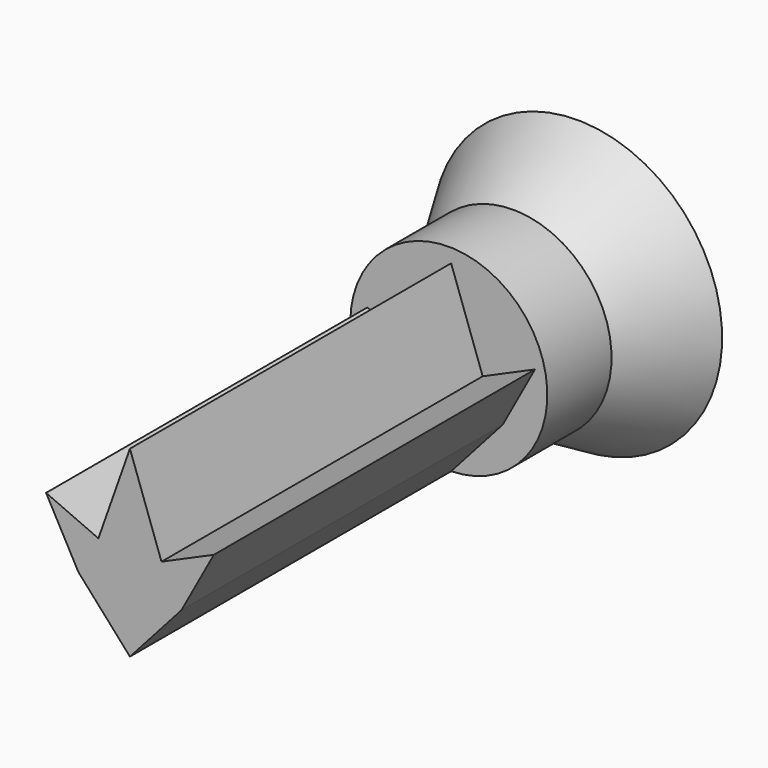
from build123d import *

# Parameters (mm, degrees)
F1_DEPTH  = 75
F3_DEPTH  = 15
F3_FACE_R = 18.3992120147
F4_DEPTH  = 15
F4_TAPER  = -30


with BuildPart() as f1:
    # F0 (on Front) → F1 (new body)
    with BuildSketch(Plane.XZ):
        Polygon((-15.2326680545, 3.4489048412), (-9.1970840294, -7.6163323829), (0.4311103548, -18.3941606665), (10.0593047391, -7.6163323829), (16.0948887642, 3.4489048412), (6.3229899097, -0.8622264722), (0.4311103548, 15.8074827632), (-5.4607692, -0.8622264722), align=None)
    extrude(amount=F1_DEPTH)


with BuildPart() as f3:
    # F2 (on face) → F3 (new body)
    with BuildSketch(Plane(origin=(0, 0, 0), x_dir=(-1, 0, 0), z_dir=(0, 1, 0))):
        with BuildLine():
            ThreePointArc((-0.4311103548, -18.3941606665), (12.8568836026, -13.161745583), (18.3992120147, 0))
            ThreePointArc((18.3992120147, 0), (-12.8568836026, 13.161745583), (-0.4311103548, -18.3941606665))
        make_face()
        Polygon((9.1970840294, -7.6163323829), (-0.4311103548, -18.3941606665), (-10.0593047391, -7.6163323829), (-16.0948887642, 3.4489048412), (-6.3229899097, -0.8622264722), (-0.4311103548, 15.8074827632), (5.4607692, -0.8622264722), (15.2326680545, 3.4489048412), align=None, mode=Mode.SUBTRACT)
        Polygon((-10.0593047391, -7.6163323829), (-0.4311103548, -18.3941606665), (9.1970840294, -7.6163323829), (15.2326680545, 3.4489048412), (5.4607692, -0.8622264722), (-0.4311103548, 15.8074827632), (-6.3229899097, -0.8622264722), (-16.0948887642, 3.4489048412), align=None)
    extrude(amount=F3_DEPTH)

    # F3_face (on face) → F4 (join)
    with BuildSketch(Plane(origin=(0, 15, 0), x_dir=(-1, 0, 0), z_dir=(0, 1, 0))):
        Circle(F3_FACE_R)
    extrude(amount=F4_DEPTH, taper=F4_TAPER)


solid = Compound([f1.part, f3.part])
